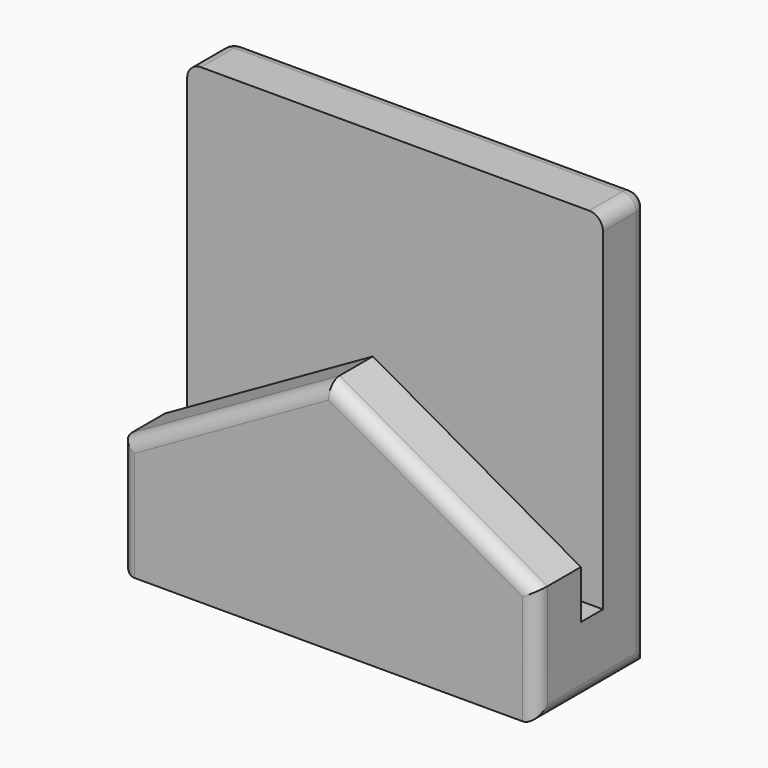
from build123d import *

# Parameters (mm, degrees)
F0_W     = 6
F0_H     = 0.8
F0_H_2   = 0.4
F1_DEPTH = 1
F2_DEPTH = 5
F3_DEPTH = 2.4
F5_DEPTH = 1
F6_R     = 0.2


with BuildPart() as f1:
    # F0 (on Top) → F1 (new body)
    with BuildSketch(Plane.XY):
        with Locations((0, -0.6)):
            Rectangle(F0_W, F0_H)
        Rectangle(F0_W, F0_H_2)
        with Locations((0, 0.6)):
            Rectangle(F0_W, F0_H)
    extrude(amount=-F1_DEPTH)

    # F0 (on Top) → F2 (join)
    with BuildSketch(Plane.XY):
        with Locations((0, 0.6)):
            Rectangle(F0_W, F0_H)
    extrude(amount=F2_DEPTH)

    # F0 (on Top) → F3 (join)
    with BuildSketch(Plane.XY):
        with Locations((0, -0.6)):
            Rectangle(F0_W, F0_H)
    extrude(amount=F3_DEPTH)

    # F4 (on face) → F5 (cut)
    with BuildSketch(Plane.XZ.offset(1)):
        Polygon((-3, 2.4), (-3, 0.7), (0, 2.4), align=None)
        Polygon((3, 2.4), (0, 2.4), (3, 0.7), align=None)
    extrude(amount=-F5_DEPTH, mode=Mode.SUBTRACT)

    # F6
    f6_edges = [f1.edges().sort_by_distance(p)[0] for p in [
        (3, 0.6, 5),
        (-3, 0.6, 5),
        (3, 0, -1),
        (-3, 0, -1),
        (3, 1, 2),
        (-3, 1, 2),
        (3, -1, -0.15),
        (-3, -1, -0.15),
        (-1.5, -1, 1.55),
        (1.5, -1, 1.55),
        (0, 1, 5),
    ]]
    fillet(f6_edges, radius=F6_R)


solid = f1.part
